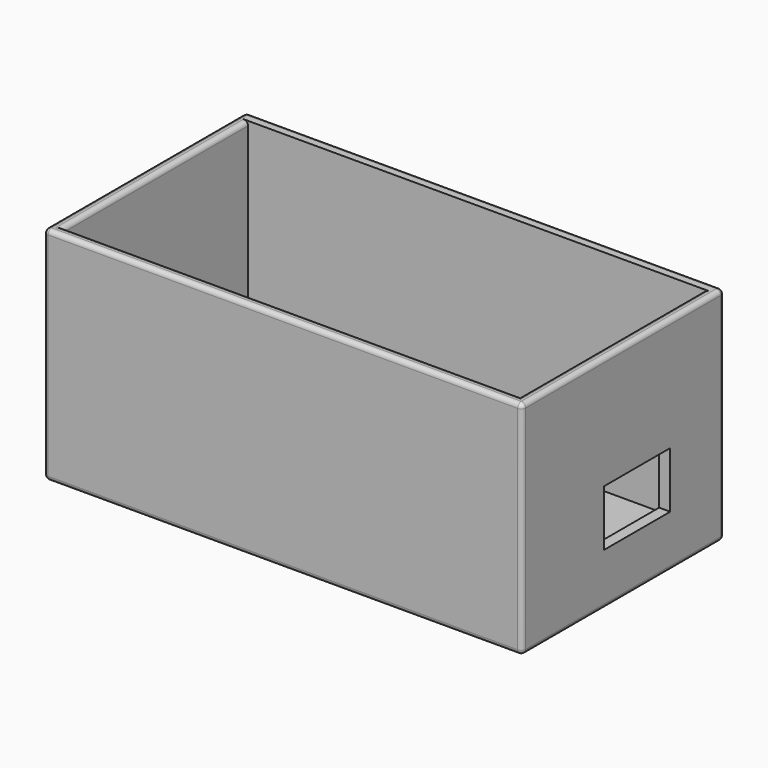
from build123d import *

# Parameters (mm, degrees)
F0_W         = 108.091738075
F0_H         = 57.078147307
F1_DEPTH     = 50
F2_T         = -2.5
F3_R         = 1
F4_T1_DEPTH  = 48
F4_T3_DEPTH  = 106.091738075
F4_T5_DEPTH  = 55.078147307
F4_S9_W      = 1
F4_S9_H      = 1
F4_T10_DEPTH = 1
F4_S15_W     = 1
F4_S15_H     = 1
F4_T16_DEPTH = 1
F4_T20_ANGLE = 90
F4_T22_ANGLE = 90
F4_T24_ANGLE = 90
F5_W         = 18.639581278
F5_H         = 12.6642128453
F6_DEPTH     = 25


# Not quite as in the source:
# - a fillet or chamfer that OpenCascade refuses, or shapes differently, is made with other operations: its cross-section is extruded or revolved along the edge and cut away or added


with BuildPart() as f1:
    # F0 (on Top) → F1 (new body)
    with BuildSketch(Plane.XY):
        with Locations((-7.7590625733, 5.3510768339)):
            Rectangle(F0_W, F0_H)
    extrude(amount=F1_DEPTH)

    # F2
    f2_openings = [f1.faces().sort_by_distance(p)[0] for p in [
        (-7.759063, 5.351077, 50),
    ]]
    offset(amount=F2_T, openings=f2_openings)

    # F3
    f3_edges = [f1.edges().sort_by_distance(p)[0] for p in [
        (-7.759063, -23.187997, 50),
        (-61.804932, -23.187997, 25),
        (-7.759063, -20.687997, 50),
        (-59.304932, 5.351077, 50),
        (-61.804932, 5.351077, 50),
        (-7.759063, -23.187997, 0),
        (46.286806, -23.187997, 25),
        (43.786806, 5.351077, 50),
        (46.286806, 5.351077, 50),
        (46.286806, 5.351077, 0),
    ]]
    fillet(f3_edges, radius=F3_R)

    # F4: fillet of radius 1 on 3 edges, made by hand

    # F4_s2 → F4_t1 (cut)
    with BuildSketch(Plane.XY.offset(1)):
        with BuildLine():
            ThreePointArc((45.2868064642, 33.8901504874), (45.9939132454, 33.5972572686), (46.2868064642, 32.8901504874))
            Line((46.2868064642, 32.8901504874), (46.2868064642, 33.8901504874))
            Line((46.2868064642, 33.8901504874), (45.2868064642, 33.8901504874))
        make_face()
        with BuildLine():
            ThreePointArc((-60.8049316108, 33.8901504874), (-61.512038392, 33.5972572686), (-61.8049316108, 32.8901504874))
            Line((-61.8049316108, 32.8901504874), (-61.8049316108, 33.8901504874))
            Line((-61.8049316108, 33.8901504874), (-60.8049316108, 33.8901504874))
        make_face()
    extrude(amount=F4_T1_DEPTH, mode=Mode.SUBTRACT)

    # F4_s4 → F4_t3 (cut)
    with BuildSketch(Plane.YZ.offset(-60.8049316108)):
        with BuildLine():
            ThreePointArc((33.8901504874, 49), (33.5972572686, 49.7071067812), (32.8901504874, 50))
            Line((32.8901504874, 50), (33.8901504874, 50))
            Line((33.8901504874, 50), (33.8901504874, 49))
        make_face()
        with BuildLine():
            ThreePointArc((33.8901504874, 1), (33.5972572686, 0.2928932188), (32.8901504874, 0))
            Line((32.8901504874, 0), (33.8901504874, 0))
            Line((33.8901504874, 0), (33.8901504874, 1))
        make_face()
    extrude(amount=F4_T3_DEPTH, mode=Mode.SUBTRACT)

    # F4_s6 → F4_t5 (cut)
    with BuildSketch(Plane.XZ.offset(-32.8901504874)):
        with BuildLine():
            ThreePointArc((-60.8049316108, 0), (-61.512038392, 0.2928932188), (-61.8049316108, 1))
            Line((-61.8049316108, 1), (-61.8049316108, 0))
            Line((-61.8049316108, 0), (-60.8049316108, 0))
        make_face()
    extrude(amount=F4_T5_DEPTH, mode=Mode.SUBTRACT)


with BuildPart() as f4_tool8:
    # F4_s9 → F4_t10 (new body)
    with BuildSketch(Plane.XY.offset(1)):
        with Locations((-61.3049316108, -22.6879968196)):
            Rectangle(F4_S9_W, F4_S9_H)
    extrude(amount=-F4_T10_DEPTH)

    # F4_s11 → F4_t12 (revolve, cut)
    with BuildSketch(Plane(origin=(-60.8049316108, -22.1879968196, 1), x_dir=(0.7071067812, 0.7071067812, 0), z_dir=(-0.7071067812, 0.7071067812, 0))):
        with BuildLine():
            ThreePointArc((0, -1), (1, 0), (0, 1))
            Line((0, 1), (0, -1))
        make_face()
    revolve(axis=Axis((-60.8049316108, -22.1879968196, 1), (0, 0, -1)), mode=Mode.SUBTRACT)


with BuildPart() as f1_1:
    add(f1.part)

    # F4_t7: cut F4_tool8
    add(f4_tool8.part, mode=Mode.SUBTRACT)


with BuildPart() as f4_tool14:
    # F4_s15 → F4_t16 (new body)
    with BuildSketch(Plane.XZ.offset(-32.8901504874)):
        with Locations((-61.3049316108, 0.5)):
            Rectangle(F4_S15_W, F4_S15_H)
    extrude(amount=-F4_T16_DEPTH)

    # F4_s17 → F4_t18 (revolve, cut)
    with BuildSketch(Plane(origin=(-60.8049316108, 32.8901504874, 1), x_dir=(0.7071067812, 0, 0.7071067812), z_dir=(-0.7071067812, 0, 0.7071067812))):
        with BuildLine():
            ThreePointArc((0, -1), (1, 0), (0, 1))
            Line((0, 1), (0, -1))
        make_face()
    revolve(axis=Axis((-60.8049316108, 32.8901504874, 1), (0, 1, 0)), mode=Mode.SUBTRACT)


with BuildPart() as f1_2:
    add(f1_1.part)

    # F4_t13: cut F4_tool14
    add(f4_tool14.part, mode=Mode.SUBTRACT)

    # F4_s19 → F4_t20 (revolve, cut)
    with BuildSketch(Plane.XY.offset(49)):
        with BuildLine():
            ThreePointArc((45.2868064642, 33.8901504874), (45.9939132454, 33.5972572686), (46.2868064642, 32.8901504874))
            Line((46.2868064642, 32.8901504874), (46.2868064642, 33.8901504874))
            Line((46.2868064642, 33.8901504874), (45.2868064642, 33.8901504874))
        make_face()
    revolve(axis=Axis((45.2868064642, 33.8901504874, 49), (0, -1, 0)), revolution_arc=F4_T20_ANGLE, mode=Mode.SUBTRACT)

    # F4_s21 → F4_t22 (revolve, cut)
    with BuildSketch(Plane.XY.offset(49)):
        with BuildLine():
            ThreePointArc((-60.8049316108, 33.8901504874), (-61.512038392, 33.5972572686), (-61.8049316108, 32.8901504874))
            Line((-61.8049316108, 32.8901504874), (-61.8049316108, 33.8901504874))
            Line((-61.8049316108, 33.8901504874), (-60.8049316108, 33.8901504874))
        make_face()
    revolve(axis=Axis((-60.8049316108, 33.8901504874, 49), (0, 1, 0)), revolution_arc=F4_T22_ANGLE, mode=Mode.SUBTRACT)

    # F4_s23 → F4_t24 (revolve, cut)
    with BuildSketch(Plane.XY.offset(1)):
        with BuildLine():
            ThreePointArc((45.2868064642, 33.8901504874), (45.9939132454, 33.5972572686), (46.2868064642, 32.8901504874))
            Line((46.2868064642, 32.8901504874), (46.2868064642, 33.8901504874))
            Line((46.2868064642, 33.8901504874), (45.2868064642, 33.8901504874))
        make_face()
    revolve(axis=Axis((45.2868064642, 33.8901504874, 1), (0, 1, 0)), revolution_arc=F4_T24_ANGLE, mode=Mode.SUBTRACT)

    # F5 (on face) → F6 (cut)
    with BuildSketch(Plane.YZ.offset(46.2868064642)):
        with Locations((9.319790639, 18.1044735946)):
            Rectangle(F5_W, F5_H)
    extrude(amount=-F6_DEPTH, mode=Mode.SUBTRACT)


solid = f1_2.part
